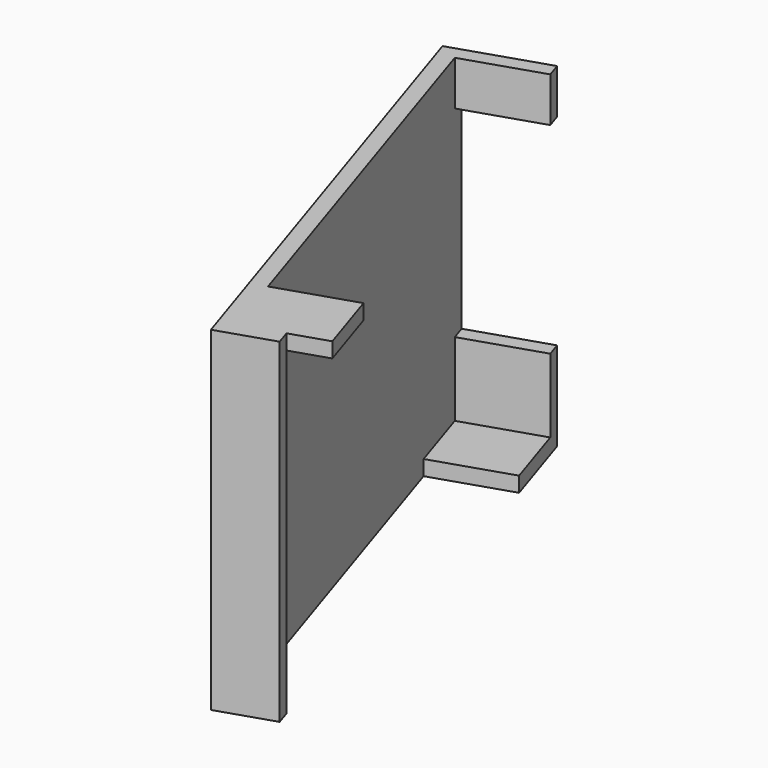
from build123d import *

# Parameters (mm, degrees)
F0_R         = 9.525
F0_R_2       = 7.9375
F1_DEPTH     = 12.7
F2_W         = 66.675
F2_H         = 102.108
F3_DEPTH     = 3.175
F5_DEPTH     = 8.255
F4_W         = 3.0118730456
F4_H         = 13.7502128413
F4_W_2       = 8.89
F4_H_2       = 3.0118730456
F6_DEPTH     = 15.875
F7_TEXT_SIZE = 10.8684896704
F8_DEPTH     = 3.175
F9_ANGLE     = 90
F10_ANGLE    = 18


# Not quite as in the source:
# - Text() gives the source's letters only with a copy of the font that has no kerning and outlines rounded to 1/6400 em; it was checked with that copy


with BuildPart() as f1:
    # F0 (on Top) → F1 (new body)
    with BuildSketch(Plane.XY):
        Circle(F0_R)
        Circle(F0_R_2, mode=Mode.SUBTRACT)
    extrude(amount=F1_DEPTH)

    # F2 (on Top) → F3 (join)
    with BuildSketch(Plane.XY):
        Rectangle(F2_W, F2_H)
    extrude(amount=-F3_DEPTH)

    # F4 (on face) → F5 (join)
    with BuildSketch(Plane(origin=(0, 0, -3.175), x_dir=(1, 0, 0), z_dir=(0, 0, -1))):
        Polygon((33.3375, 51.054), (-33.3375, 51.054), (-33.3375, 48.0421269544), (30.3256269544, 48.0421269544), (33.3375, 48.0421269544), align=None)
    extrude(amount=F5_DEPTH)

    # F4 (on face) → F6 (join)
    with BuildSketch(Plane(origin=(0, 0, -3.175), x_dir=(1, 0, 0), z_dir=(0, 0, -1))):
        with Locations((-31.8315634772, -41.1670205338)):
            Rectangle(F4_W, F4_H)
        Polygon((-30.3256269544, -48.0421269544), (-33.3375, -48.0421269544), (-33.3375, -51.054), (-15.6400557607, -51.054), (-15.6400557607, -48.0421269544), align=None)
        with Locations((31.8315634772, 41.1670205338)):
            Rectangle(F4_W, F4_H)
        with Locations((28.8925, -49.5480634772)):
            Rectangle(F4_W_2, F4_H_2)
    extrude(amount=F6_DEPTH)

    # F7 (on face) → F8 (join)
    with BuildSketch(Plane.XY):
        with Locations(Location((25.4, -21.2762604196), (0, 0, 180))):
            Text('EMOTERS', F7_TEXT_SIZE, font='Open Sans', font_style=FontStyle.BOLD, text_align=(TextAlign.LEFT, TextAlign.BOTTOM))
    extrude(amount=F8_DEPTH)


with BuildPart() as f1_1:
    # F9: moved
    add(f1.part.rotate(Axis((-33.3375, 0, 0), (0, -1, 0)), F9_ANGLE))


with BuildPart() as f1_2:
    # F10: moved
    add(f1_1.part.rotate(Axis((-33.3375, -51.054, 33.3375), (0, 0, 1)), F10_ANGLE))


solid = f1_2.part
